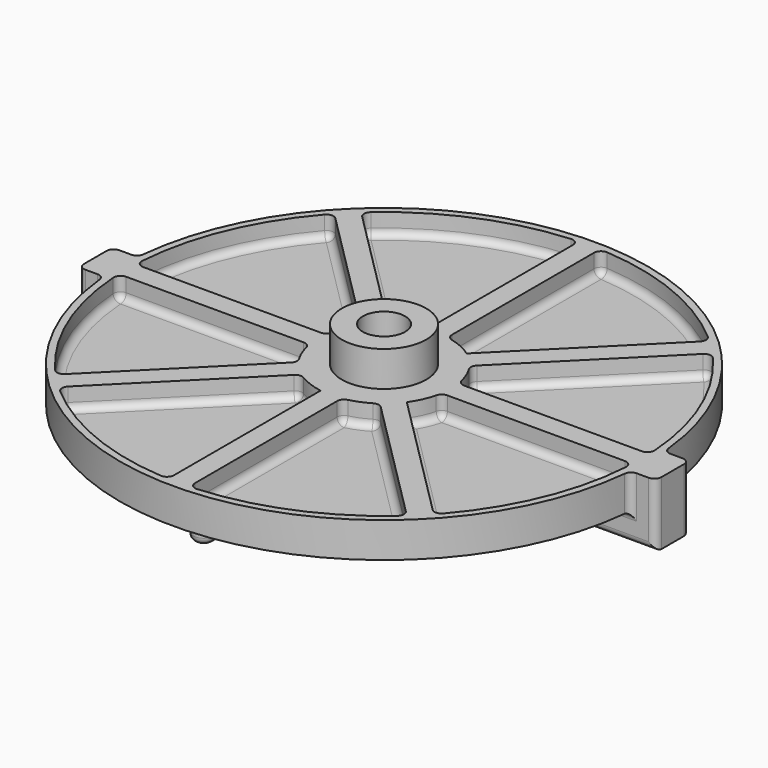
from build123d import *

# Parameters (mm, degrees)
F0_R      = 37.5
F1_DEPTH  = 5
F3_DEPTH  = 3
F4_W      = 82
F4_H      = 6
F5_DEPTH  = 4
F7_DEPTH  = 5
F8_R      = 1
F10_DEPTH = 4
F11_R     = 1
F12_R     = 6
F13_DEPTH = 5
F15_D     = 6
F15_DEPTH = 8
F15_TIP   = 1.8025818571
F16_R     = 1


with BuildPart() as f1:
    # F0 (on Top) → F1 (new body)
    with BuildSketch(Plane.XY):
        Circle(F0_R)
    extrude(amount=F1_DEPTH)

    # F2 (on face) → F3 (cut)
    with BuildSketch(Plane.XY.offset(5)):
        with BuildLine():
            ThreePointArc((-26.1006282229, 23.9793078793), (-26.8429681472, 24.2715802182), (-27.562882469, 23.9277560586))
            ThreePointArc((-27.562882469, 23.9277560586), (-33.7216029367, 13.9679452813), (-36.4093796705, 2.5704225352))
            ThreePointArc((-36.4093796705, 2.5704225352), (-36.1434437665, 1.8182458417), (-35.4118624193, 1.5))
            Line((-35.4118624193, 1.5), (-10.1980390272, 1.5))
            ThreePointArc((-10.1980390272, 1.5), (-9.5808256273, 1.7132042075), (-9.2267972151, 2.2619047619))
            ThreePointArc((-9.2267972151, 2.2619047619), (-8.7768555589, 3.6354926075), (-8.123739075, 4.9249226839))
            ThreePointArc((-8.123739075, 4.9249226839), (-7.9860850832, 5.5632484578), (-8.2717627227, 6.1504423791))
            Line((-8.2717627227, 6.1504423791), (-26.1006282229, 23.9793078793))
        make_face()
        with BuildLine():
            ThreePointArc((8.123739075, 4.9249226839), (8.7768555589, 3.6354926075), (9.2267972151, 2.2619047619))
            ThreePointArc((9.2267972151, 2.2619047619), (9.5808256273, 1.7132042075), (10.1980390272, 1.5))
            Line((10.1980390272, 1.5), (35.4118624193, 1.5))
            ThreePointArc((35.4118624193, 1.5), (36.1434437665, 1.8182458417), (36.4093796705, 2.5704225352))
            ThreePointArc((36.4093796705, 2.5704225352), (33.7216029367, 13.9679452813), (27.562882469, 23.9277560586))
            ThreePointArc((27.562882469, 23.9277560586), (26.8429681472, 24.2715802182), (26.1006282229, 23.9793078793))
            Line((26.1006282229, 23.9793078793), (8.2717627227, 6.1504423791))
            ThreePointArc((8.2717627227, 6.1504423791), (7.9860850832, 5.5632484578), (8.123739075, 4.9249226839))
        make_face()
        with BuildLine():
            Line((1.5, 35.4118624193), (1.5, 10.1980390272))
            ThreePointArc((1.5, 10.1980390272), (1.7132042075, 9.5808256273), (2.2619047619, 9.2267972151))
            ThreePointArc((2.2619047619, 9.2267972151), (3.991523609, 8.6207737053), (5.5725894089, 7.6939097525))
            Line((5.5725894089, 7.6939097525), (23.9793078793, 26.1006282229))
            ThreePointArc((23.9793078793, 26.1006282229), (24.2715802182, 26.8429681472), (23.9277560586, 27.562882469))
            ThreePointArc((23.9277560586, 27.562882469), (13.9679452813, 33.7216029367), (2.5704225352, 36.4093796705))
            ThreePointArc((2.5704225352, 36.4093796705), (1.8182458417, 36.1434437665), (1.5, 35.4118624193))
        make_face()
        with BuildLine():
            ThreePointArc((-2.2619047619, 9.2267972151), (-1.7132042075, 9.5808256273), (-1.5, 10.1980390272))
            Line((-1.5, 10.1980390272), (-1.5, 35.4118624193))
            ThreePointArc((-1.5, 35.4118624193), (-1.8182458417, 36.1434437665), (-2.5704225352, 36.4093796705))
            ThreePointArc((-2.5704225352, 36.4093796705), (-13.9679452813, 33.7216029367), (-23.9277560586, 27.562882469))
            ThreePointArc((-23.9277560586, 27.562882469), (-24.2715802182, 26.8429681472), (-23.9793078793, 26.1006282229))
            Line((-23.9793078793, 26.1006282229), (-6.1504423791, 8.2717627227))
            ThreePointArc((-6.1504423791, 8.2717627227), (-5.5632484578, 7.9860850832), (-4.9249226839, 8.123739075))
            ThreePointArc((-4.9249226839, 8.123739075), (-3.6354926075, 8.7768555589), (-2.2619047619, 9.2267972151))
        make_face()
        with BuildLine():
            ThreePointArc((-9.2267972151, -2.2619047619), (-9.5808256273, -1.7132042075), (-10.1980390272, -1.5))
            Line((-10.1980390272, -1.5), (-35.4118624193, -1.5))
            ThreePointArc((-35.4118624193, -1.5), (-36.1434437665, -1.8182458417), (-36.4093796705, -2.5704225352))
            ThreePointArc((-36.4093796705, -2.5704225352), (-33.7216029367, -13.9679452813), (-27.562882469, -23.9277560586))
            ThreePointArc((-27.562882469, -23.9277560586), (-26.8429681472, -24.2715802182), (-26.1006282229, -23.9793078793))
            Line((-26.1006282229, -23.9793078793), (-8.2717627227, -6.1504423791))
            ThreePointArc((-8.2717627227, -6.1504423791), (-7.9860850832, -5.5632484578), (-8.123739075, -4.9249226839))
            ThreePointArc((-8.123739075, -4.9249226839), (-8.7768555589, -3.6354926075), (-9.2267972151, -2.2619047619))
        make_face()
        with BuildLine():
            ThreePointArc((-4.9249226839, -8.123739075), (-5.5632484578, -7.9860850832), (-6.1504423791, -8.2717627227))
            Line((-6.1504423791, -8.2717627227), (-23.9793078793, -26.1006282229))
            ThreePointArc((-23.9793078793, -26.1006282229), (-24.2715802182, -26.8429681472), (-23.9277560586, -27.562882469))
            ThreePointArc((-23.9277560586, -27.562882469), (-13.9679452813, -33.7216029367), (-2.5704225352, -36.4093796705))
            ThreePointArc((-2.5704225352, -36.4093796705), (-1.8182458417, -36.1434437665), (-1.5, -35.4118624193))
            Line((-1.5, -35.4118624193), (-1.5, -9.3808315196))
            ThreePointArc((-1.5, -9.3808315196), (-3.2733741349, -8.9182409573), (-4.9249226839, -8.123739075))
        make_face()
        with BuildLine():
            ThreePointArc((2.2619047619, -9.2267972151), (1.7132042075, -9.5808256273), (1.5, -10.1980390272))
            Line((1.5, -10.1980390272), (1.5, -35.4118624193))
            ThreePointArc((1.5, -35.4118624193), (1.8182458417, -36.1434437665), (2.5704225352, -36.4093796705))
            ThreePointArc((2.5704225352, -36.4093796705), (13.9679452813, -33.7216029367), (23.9277560586, -27.562882469))
            ThreePointArc((23.9277560586, -27.562882469), (24.2715802182, -26.8429681472), (23.9793078793, -26.1006282229))
            Line((23.9793078793, -26.1006282229), (6.1504423791, -8.2717627227))
            ThreePointArc((6.1504423791, -8.2717627227), (5.5632484578, -7.9860850832), (4.9249226839, -8.123739075))
            ThreePointArc((4.9249226839, -8.123739075), (3.6354926075, -8.7768555589), (2.2619047619, -9.2267972151))
        make_face()
        with BuildLine():
            ThreePointArc((9.2267972151, -2.2619047619), (8.6207737053, -3.991523609), (7.6939097525, -5.5725894089))
            Line((7.6939097525, -5.5725894089), (26.1006282229, -23.9793078793))
            ThreePointArc((26.1006282229, -23.9793078793), (26.8429681472, -24.2715802182), (27.562882469, -23.9277560586))
            ThreePointArc((27.562882469, -23.9277560586), (33.7216029367, -13.9679452813), (36.4093796705, -2.5704225352))
            ThreePointArc((36.4093796705, -2.5704225352), (36.1434437665, -1.8182458417), (35.4118624193, -1.5))
            Line((35.4118624193, -1.5), (10.1980390272, -1.5))
            ThreePointArc((10.1980390272, -1.5), (9.5808256273, -1.7132042075), (9.2267972151, -2.2619047619))
        make_face()
    extrude(amount=-F3_DEPTH, mode=Mode.SUBTRACT)

    # F4 (on face) → F5 (join)
    with BuildSketch(Plane(origin=(0, 0, 0), x_dir=(1, 0, 0), z_dir=(0, 0, -1))):
        Rectangle(F4_W, F4_H)
    extrude(amount=F5_DEPTH)

    # F6 (on face) → F7 (join, through all)
    with BuildSketch(Plane.XY):
        with BuildLine():
            Line((-37.3798073831, 3), (-41, 3))
            Line((-41, 3), (-41, -3))
            Line((-41, -3), (-37.3798073831, -3))
            ThreePointArc((-37.3798073831, -3), (-37.4785818612, 0), (-37.3798073831, 3))
        make_face()
        with BuildLine():
            Line((37.3798073831, -3), (41, -3))
            Line((41, -3), (41, 3))
            Line((41, 3), (37.3798073831, 3))
            ThreePointArc((37.3798073831, 3), (37.4785818612, 0), (37.3798073831, -3))
        make_face()
    extrude(amount=F7_DEPTH)

    # F8
    f8_edges = [f1.edges().sort_by_distance(p)[0] for p in [
        (-41, 3, 0.5),
        (-41, -3, 0.5),
        (41, -3, 0.5),
        (41, 3, 0.5),
        (0, 3, -4),
        (0, -3, -4),
        (0, 3, 0),
        (0, -3, 0),
        (-37.379807, -3, 2.5),
        (-37.379807, 3, 2.5),
        (37.379807, 3, 2.5),
        (37.379807, -3, 2.5),
    ]]
    fillet(f8_edges, radius=F8_R)

    # F9 (on face) → F10 (join)
    with BuildSketch(Plane(origin=(0, 0, 0), x_dir=(1, 0, 0), z_dir=(0, 0, -1))):
        with BuildLine():
            ThreePointArc((1.5, 32), (0, 33.5), (-1.5, 32))
            Line((-1.5, 32), (-1.5, 17))
            ThreePointArc((-1.5, 17), (0, 15.5), (1.5, 17))
            Line((1.5, 17), (1.5, 32))
        make_face()
        with BuildLine():
            Line((-1.5, -17), (-1.5, -32))
            ThreePointArc((-1.5, -32), (0, -33.5), (1.5, -32))
            Line((1.5, -32), (1.5, -17))
            ThreePointArc((1.5, -17), (0, -15.5), (-1.5, -17))
        make_face()
    extrude(amount=F10_DEPTH)

    # F11
    f11_edges = [f1.edges().sort_by_distance(p)[0] for p in [
        (1.5, -24.5, -4),
        (-1.5, -24.5, -4),
        (-1.5, 24.5, -4),
        (0, 33.5, -4),
        (1.5, 24.5, -4),
        (0, 15.5, -4),
    ]]
    fillet(f11_edges, radius=F11_R)

    # F12 (on face) → F13 (join)
    with BuildSketch(Plane.XY.offset(5)):
        Circle(F12_R)
    extrude(amount=F13_DEPTH)

    # F15
    with Locations(Plane.XY.offset(10)):
        with Locations((0, 0)):
            Hole(F15_D / 2, depth=F15_DEPTH)
            with Locations((0, 0, -(F15_DEPTH + F15_TIP / 2))):  # 118° drill point
                Cone(0, F15_D / 2, F15_TIP, mode=Mode.SUBTRACT)

    # F16
    f16_edges = [f1.edges().sort_by_distance(p)[0] for p in [
        (-22.804951, -1.5, 2),
        (-33.721603, 13.967945, 2),
        (-13.967945, 33.721603, 2),
        (1.5, 22.804951, 2),
        (17.186195, 15.064875, 2),
        (13.967945, 33.721603, 2),
        (1.818246, 36.143444, 2),
        (14.775949, 16.897269, 2),
        (16.897269, -14.775949, 2),
        (26.842968, -24.27158, 2),
        (33.721603, -13.967945, 2),
        (36.143444, -1.818246, 2),
        (22.804951, -1.5, 2),
        (9.580826, -1.713204, 2),
        (8.620774, -3.991524, 2),
        (15.064875, -17.186195, 2),
        (-1.5, -22.396347, 2),
    ]]
    fillet(f16_edges, radius=F16_R)


solid = f1.part
